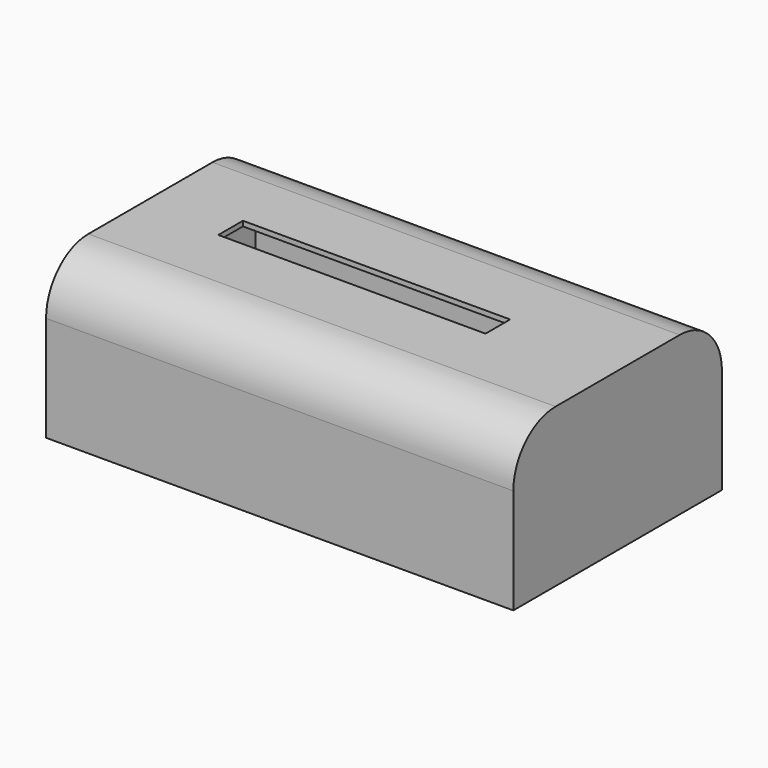
from build123d import *

# Parameters (mm, degrees)
F0_W     = 238.8670668006
F0_H     = 133.2817673683
F1_DEPTH = 80.772
F2_R     = 26.9812507731
F3_W     = 136.5834623575
F3_H     = 15.7284336165
F4_DEPTH = 15.748
F5_T     = 2.54


# Not quite as in the source:
# - a shell that OpenCascade refuses in one call is made with other operations: the cavity is built on its own and cut out


with BuildPart() as f1:
    # F0 (on Top) → F1 (new body)
    with BuildSketch(Plane.XY):
        with Locations((2.9073394835, 0.8117333055)):
            Rectangle(F0_W, F0_H)
    extrude(amount=F1_DEPTH)

    # F2
    f2_edges = [f1.edges().sort_by_distance(p)[0] for p in [
        (2.907339, -65.82915, 80.772),
        (2.907339, 67.452617, 80.772),
    ]]
    fillet(f2_edges, radius=F2_R)

    # F3 (on face) → F4 (join)
    with BuildSketch(Plane.XY.offset(80.772)):
        with Locations((-7.1703717113, 0.7790052332)):
            Rectangle(F3_W, F3_H)
    extrude(amount=F4_DEPTH)

    # F5: shell of thickness 2.54, made by hand


with BuildPart() as f5_core1:
    # F5_t2: copy of F1
    add(f1.part)

    # the walls: a layer under each face that stays
    f5_faces = [f5_core1.faces().sort_by_distance(p)[0] for p in [
        (2.9073394835, 67.4526169896, 26.8953746135),
        (122.3408728838, 0.8117333055, 40.386),
        (2.9073394835, 59.5499916031, 72.8693746135),
        (2.9073394835, 0.8117333055, 0),
        (-116.5261939168, 0.8117333055, 40.386),
        (2.9073394835, -65.8291503787, 26.8953746135),
        (2.9073394835, -57.9265249922, 72.8693746135),
        (-76.7150161167, -25.6280219686, 80.772),
    ]]
    thicken(f5_faces, amount=-F5_T, mode=Mode.SUBTRACT)


with BuildPart() as f1_1:
    add(f1.part)

    # what is left inside the walls is the cavity
    f5_cavity = [f5_core1.part.solids().sort_by_distance(p)[0] for p in [
        (2.907339, -20.555228, 2.5654),
    ]]
    add(f5_cavity, mode=Mode.SUBTRACT)


solid = f1_1.part
